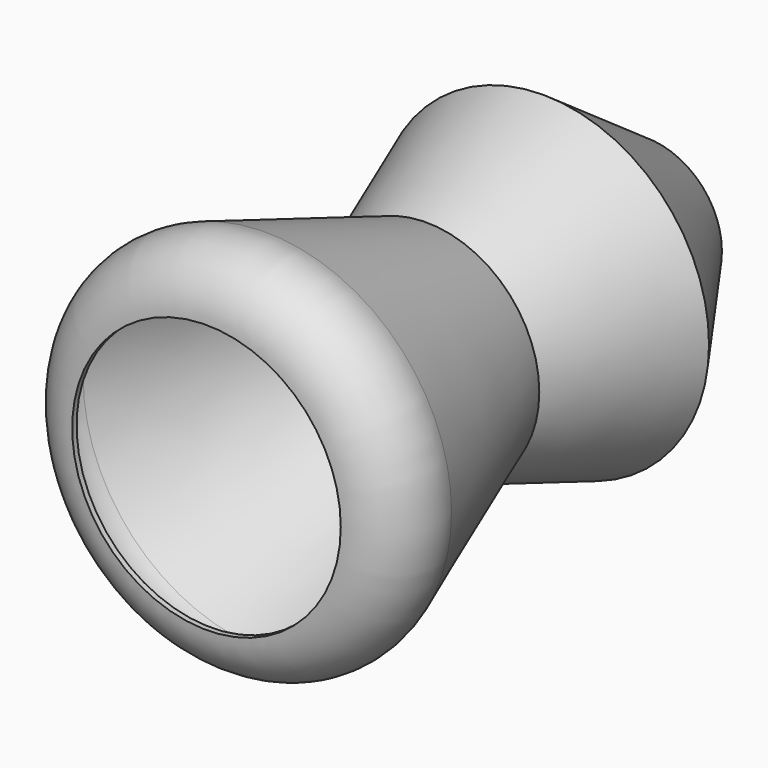
from build123d import *

# Parameters (mm, degrees)
F0_R     = 52.0623730702
F1_DEPTH = 127
F1_TAPER = -20
F2_R     = 25.4
F3_SIZE  = 63.5
F4_T     = -2.54


# Not quite as in the source:
# - a shell that OpenCascade refuses in one call is made with other operations: the cavity is built on its own and cut out


with BuildPart() as f1:
    # F0 (on Front) → F1 (new body, symmetric)
    with BuildSketch(Plane.XZ):
        Circle(F0_R)
    extrude(amount=F1_DEPTH, both=True, taper=F1_TAPER)

    # F2
    f2_edges = [f1.edges().sort_by_distance(p)[0] for p in [
        (-98.286593, -127, 0),
    ]]
    fillet(f2_edges, radius=F2_R)

    # F3
    f3_edges = [f1.edges().sort_by_distance(p)[0] for p in [
        (-98.286593, 127, 0),
    ]]
    chamfer(f3_edges, length=F3_SIZE)

    # F4: a shell. OpenCascade refuses it in one call, so the cavity is built on its own and cut out:
    # the body offset inwards by the wall thickness, plus a prism from it out through each open face.
    f4_core = offset(f1.part, amount=F4_T, kind=Kind.INTERSECTION, mode=Mode.PRIVATE)
    f4_exits = [f4_core.faces().sort_by_distance(p)[0] for p in [
        (0, -124.46, 0),
    ]]
    add(f4_core, mode=Mode.SUBTRACT)
    extrude(f4_exits, amount=-F4_T, mode=Mode.SUBTRACT)


solid = f1.part
